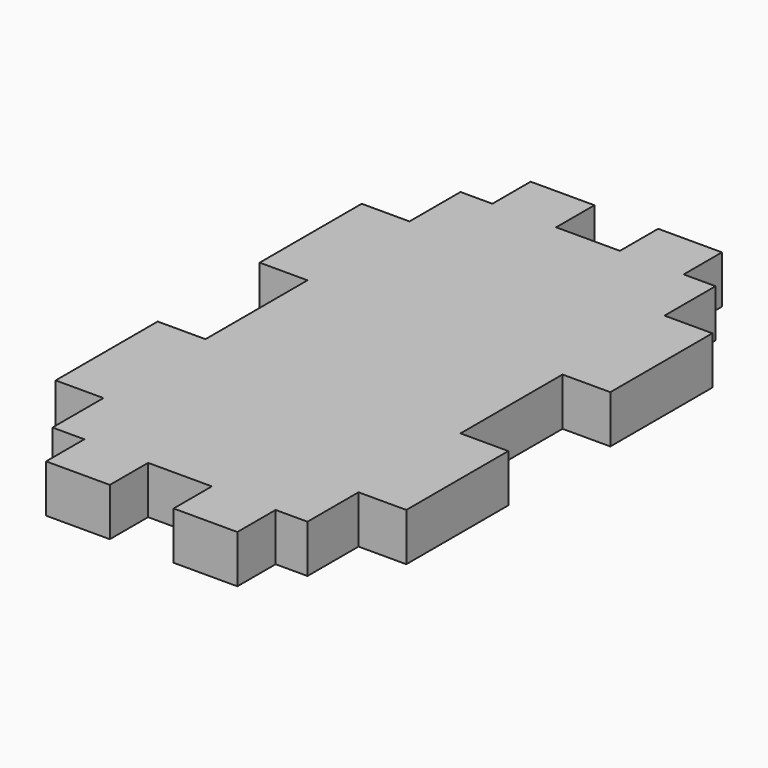
from build123d import *

# Parameters (mm, degrees)
F0_W     = 19.05
F0_H     = 50.8
F0_W_2   = 25.4
F0_H_2   = 19.05
F1_DEPTH = 19.05


# Not quite as in the source:
# - a feature names something its author has since deleted; it is built from what else it names


with BuildPart() as f1:
    # F0 (on Top) → F1 (new body)
    with BuildSketch(Plane.XY):
        with Locations((-25.5773371266, 60.6874149844)):
            Rectangle(F0_W, F0_H)
        Polygon((-3.3523371266, 111.4874149844), (-16.0523371266, 111.4874149844), (-16.0523371266, 86.0874149844), (-16.0523371266, 35.2874149844), (-16.0523371266, -15.5125850156), (-16.0523371266, -32.8271351755), (-16.0523371266, -66.3125850156), (-16.0523371266, -91.7125850156), (-3.3523371266, -91.7125850156), (22.0476628734, -91.7125850156), (47.4476628734, -91.7125850156), (72.8476628734, -91.7125850156), (85.5476628734, -91.7125850156), (85.5476628734, -66.3125850156), (85.5476628734, -15.5125850156), (85.5476628734, 35.2874149844), (85.5476628734, 86.0874149844), (85.5476628734, 111.4874149844), (72.8476628734, 111.4874149844), (47.4476628734, 111.4874149844), (22.0476628734, 111.4874149844), align=None)
        Polygon((-16.0523371266, -32.8271351755), (-16.0523371266, -15.5125850156), (-35.1023371266, -15.5125850156), (-35.1023371266, -66.3125850156), (-16.0523371266, -66.3125850156), align=None)
        with Locations((9.3476628734, -101.2375850156)):
            Rectangle(F0_W_2, F0_H_2)
        with Locations((60.1476628734, -101.2375850156)):
            Rectangle(F0_W_2, F0_H_2)
        with Locations((95.0726628734, -40.9125850156)):
            Rectangle(F0_W, F0_H)
        with Locations((95.0726628734, 60.6874149844)):
            Rectangle(F0_W, F0_H)
        with Locations((60.1476628734, 121.0124149844)):
            Rectangle(F0_W_2, F0_H_2)
        with Locations((9.3476628734, 121.0124149844)):
            Rectangle(F0_W_2, F0_H_2)
    extrude(amount=F1_DEPTH)


solid = f1.part
